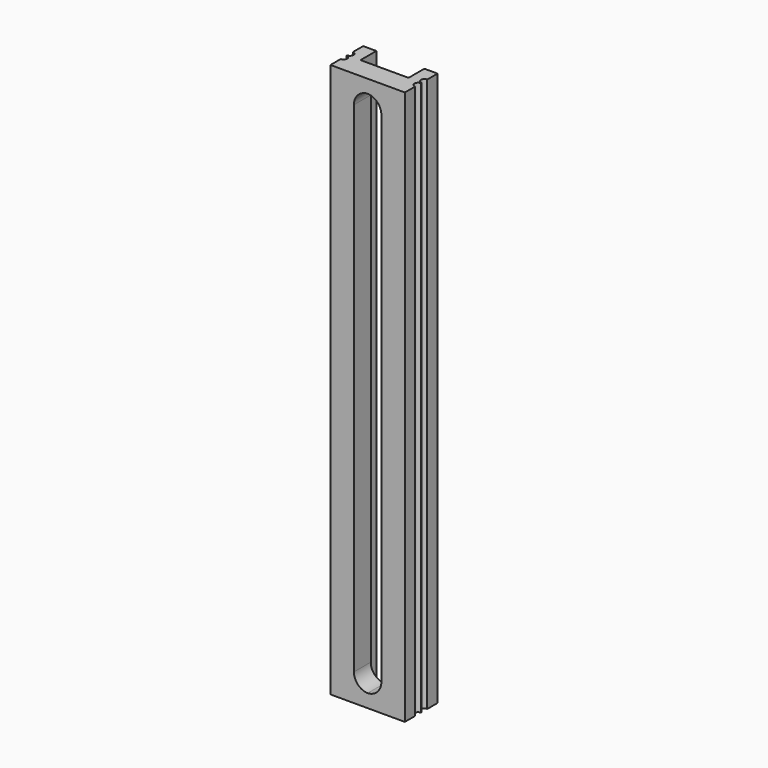
from build123d import *

# Parameters (mm, degrees)
F0_W        = 11.557
F0_H        = 133.35
F0_W_2      = 6.604
F0_H_2      = 127
F0_W_3      = 3.175
F1_DEPTH    = 5.08
F2_T1_DEPTH = 5.08
F3_DEPTH    = 4.7625
F5_DEPTH    = 133.351


# Not quite as in the source:
# - a fillet or chamfer that OpenCascade refuses, or shapes differently, is made with other operations: its cross-section is extruded or revolved along the edge and cut away or added


with BuildPart() as f1:
    # F0 (on Front) → F1 (new body)
    with BuildSketch(Plane.XZ):
        Rectangle(F0_W, F0_H)
        Rectangle(F0_W_2, F0_H_2, mode=Mode.SUBTRACT)
        with Locations((-7.366, 0)):
            Rectangle(F0_W_3, F0_H)
        with Locations((7.366, 0)):
            Rectangle(F0_W_3, F0_H)
    extrude(amount=F1_DEPTH)

    # F2: fillet of radius 3.429 on 4 edges, made by hand

    # F2_s2 → F2_t1 (join)
    with BuildSketch(Plane.XZ):
        with BuildLine():
            ThreePointArc((-0.127, 63.5), (2.2976691527, 62.4956691527), (3.302, 60.071))
            Line((3.302, 60.071), (3.302, 63.5))
            Line((3.302, 63.5), (-0.127, 63.5))
        make_face()
        with BuildLine():
            ThreePointArc((-3.302, 60.071), (-2.2976691527, 62.4956691527), (0.127, 63.5))
            Line((0.127, 63.5), (-3.302, 63.5))
            Line((-3.302, 63.5), (-3.302, 60.071))
        make_face()
        with BuildLine():
            ThreePointArc((0.127, -63.5), (-2.2976691527, -62.4956691527), (-3.302, -60.071))
            Line((-3.302, -60.071), (-3.302, -63.5))
            Line((-3.302, -63.5), (0.127, -63.5))
        make_face()
        with BuildLine():
            ThreePointArc((-0.127, -63.5), (2.2976691527, -62.4956691527), (3.302, -60.071))
            Line((3.302, -60.071), (3.302, -63.5))
            Line((3.302, -63.5), (-0.127, -63.5))
        make_face()
    extrude(amount=F2_T1_DEPTH)

    # F0 (on Front) → F3 (join)
    with BuildSketch(Plane.XZ):
        with Locations((7.366, 0)):
            Rectangle(F0_W_3, F0_H)
        with Locations((-7.366, 0)):
            Rectangle(F0_W_3, F0_H)
    extrude(amount=-F3_DEPTH)

    # F4 (on face) → F5 (cut, through all)
    with BuildSketch(Plane.XY.offset(66.675)):
        with BuildLine():
            ThreePointArc((-8.9535, -0.06985), (-8.3428425838, 0.1830925838), (-8.0899, 0.79375))
            ThreePointArc((-8.0899, 0.79375), (-8.3428425838, 1.4044074162), (-8.9535, 1.65735))
            Line((-8.9535, 1.65735), (-8.9535, -0.06985))
        make_face()
        with BuildLine():
            ThreePointArc((-8.0899, -1.11125), (-8.3428425838, -0.5005925838), (-8.9535, -0.24765))
            Line((-8.9535, -0.24765), (-8.9535, -1.97485))
            ThreePointArc((-8.9535, -1.97485), (-8.3428425838, -1.7219074162), (-8.0899, -1.11125))
        make_face()
        with BuildLine():
            ThreePointArc((8.9535, -0.24765), (8.0899, -1.11125), (8.9535, -1.97485))
            Line((8.9535, -1.97485), (8.9535, -0.24765))
        make_face()
        with BuildLine():
            Line((8.9535, -0.06985), (8.9535, 1.65735))
            ThreePointArc((8.9535, 1.65735), (8.0899, 0.79375), (8.9535, -0.06985))
        make_face()
    extrude(amount=-F5_DEPTH, mode=Mode.SUBTRACT)


solid = f1.part
